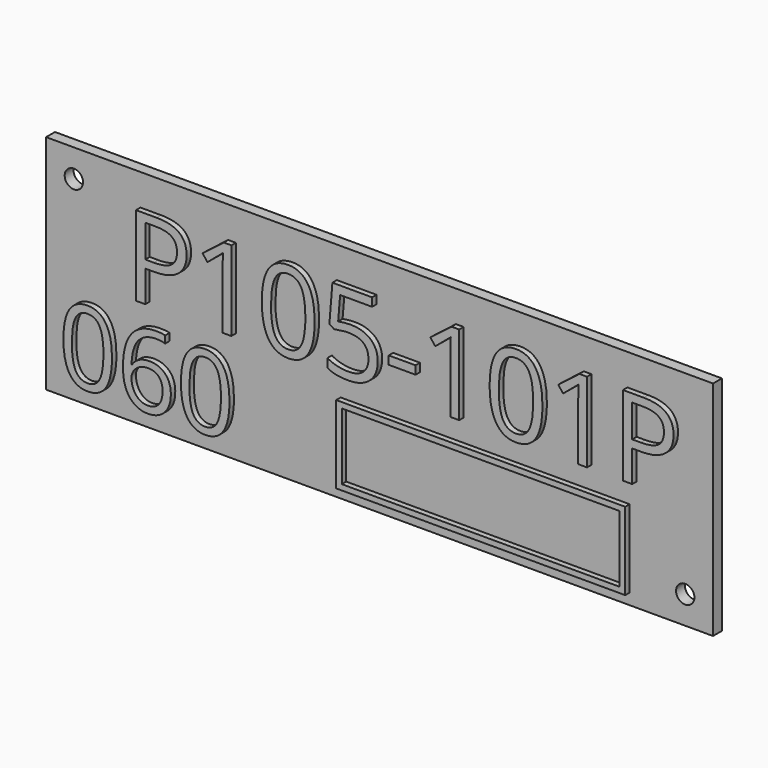
from build123d import *

# Parameters (mm, degrees)
F0_W         = 120
F0_H         = 40
F1_DEPTH     = 2
F3_D         = 3.3
F4_TEXT_SIZE = 20.1219895617
F5_DEPTH     = 1
F6_TEXT_SIZE = 18.4937691891
F7_DEPTH     = 1
F8_W         = 52
F8_H         = 14
F8_W_2       = 49.99999962
F8_H_2       = 11.99999962
F9_DEPTH     = 1


# Not quite as in the source:
# - Text() gives the source's letters only with a copy of the font that has no kerning and outlines rounded to 1/6400 em; it was checked with that copy


with BuildPart() as f1:
    # F0 (on Front) → F1 (new body)
    with BuildSketch(Plane.XZ):
        Rectangle(F0_W, F0_H)
    extrude(amount=F1_DEPTH)

    # F3 (through all)
    with Locations(Plane.XZ.offset(2)):
        with Locations((-55, 15), (55, -15)):
            Hole(F3_D / 2)

    # F4 (on face) → F5 (join)
    with BuildSketch(Plane.XZ.offset(2)):
        with Locations((-45, 0)):
            Text('P105-101P', F4_TEXT_SIZE, font='Open Sans', text_align=(TextAlign.LEFT, TextAlign.BOTTOM))
    extrude(amount=F5_DEPTH)

    # F6 (on face) → F7 (join)
    with BuildSketch(Plane.XZ.offset(2)):
        with Locations((-57, -17)):
            Text('060', F6_TEXT_SIZE, font='Open Sans', text_align=(TextAlign.LEFT, TextAlign.BOTTOM))
    extrude(amount=F7_DEPTH)

    # F8 (on face) → F9 (join)
    with BuildSketch(Plane.XZ.offset(2)):
        with Locations((19, -11)):
            Rectangle(F8_W, F8_H)
        with Locations((19, -11)):
            Rectangle(F8_W_2, F8_H_2, mode=Mode.SUBTRACT)
    extrude(amount=F9_DEPTH)


solid = f1.part
